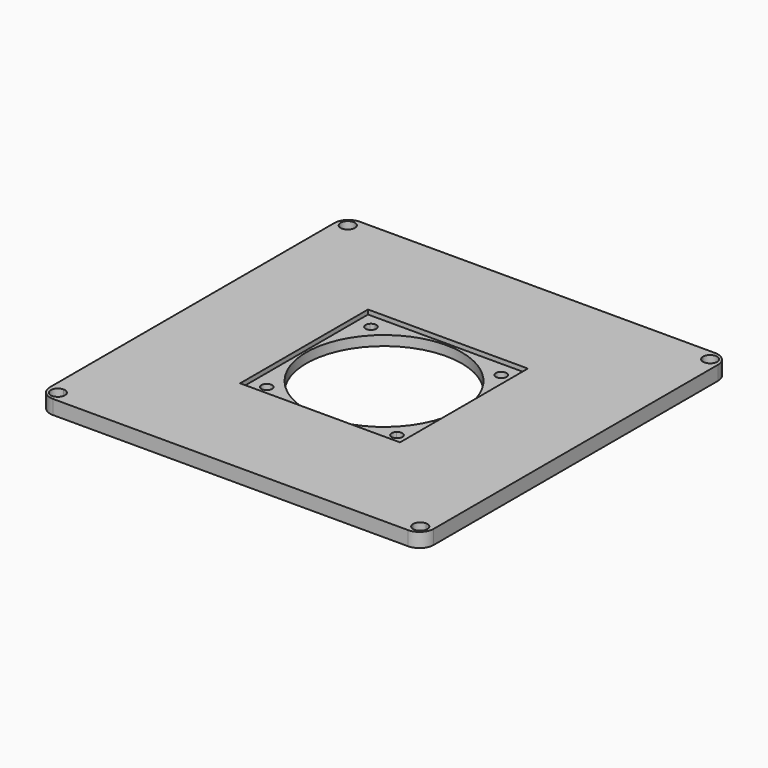
from build123d import *

# Parameters (mm, degrees)
F0_W             = 137.16
F0_H             = 137.16
F1_DEPTH         = 5.08
F2_R             = 5.08
F3_R             = 27.78125
F4_DEPTH         = 5.08
F5_W             = 57.15
F5_H             = 57.15
F6_DEPTH         = 1.5875
F8_DEPTH         = 3.4925
F8_COPIES_COUNT  = 4
F11_DEPTH        = 1.27
F11_COPIES_COUNT = 4
F13_DEPTH        = 5.08


# Not quite as in the source:
# - a pattern or mirror of a feature is missing from the dataset's text; its kind, count and spacing are read off the source's solid


with BuildPart() as f1:
    # F0 (on Top) → F1 (new body)
    with BuildSketch(Plane.XY):
        Rectangle(F0_W, F0_H)
    extrude(amount=F1_DEPTH)

    # F2
    f2_edges = [f1.edges().sort_by_distance(p)[0] for p in [
        (-68.58, -68.58, 2.54),
        (68.58, -68.58, 2.54),
        (68.58, 68.58, 2.54),
        (-68.58, 68.58, 2.54),
    ]]
    fillet(f2_edges, radius=F2_R)

    # F3 (on face) → F4 (cut, through all)
    with BuildSketch(Plane.XY.offset(5.08)):
        Circle(F3_R)
    extrude(amount=-F4_DEPTH, mode=Mode.SUBTRACT)

    # F5 (on face) → F6 (cut)
    with BuildSketch(Plane.XY.offset(5.08)):
        Rectangle(F5_W, F5_H)
    extrude(amount=-F6_DEPTH, mode=Mode.SUBTRACT)

    # F7 (on face) → F8 (cut, through all)
    with BuildSketch(Plane.XY.offset(3.4925)):
        with BuildLine():
            Line((21.9296104704, 21.9296104704), (24.6236873067, 24.6236873067))
            ThreePointArc((24.6236873067, 24.6236873067), (21.9296104704, 24.6236873067), (21.9296104704, 21.9296104704))
        make_face()
        with BuildLine():
            ThreePointArc((25.1816488886, 23.2766488886), (25.036639398, 24.0056608272), (24.6236873067, 24.6236873067))
            Line((24.6236873067, 24.6236873067), (21.9296104704, 21.9296104704))
            ThreePointArc((21.9296104704, 21.9296104704), (24.0056608272, 21.5166583791), (25.1816488886, 23.2766488886))
        make_face()
    f8 = extrude(amount=-F8_DEPTH, mode=Mode.SUBTRACT)

    # F8_copies: F8 ×4 about axis
    f8_copies_axis = Axis((0, 0, 0), (0, 0, 1))
    for i in range(1, F8_COPIES_COUNT):
        add(f8.rotate(f8_copies_axis, i * 360 / F8_COPIES_COUNT), mode=Mode.SUBTRACT)

    # F10 (on face) → F11 (cut)
    with BuildSketch(Plane(origin=(0, 0, 0), x_dir=(1, 0, 0), z_dir=(0, 0, -1))):
        Polygon((27.0866488886, 23.2766488886), (25.1816488886, 26.576205677), (21.3716488886, 26.576205677), (19.4666488886, 23.2766488886), (21.3716488886, 19.9770921002), (25.1816488886, 19.9770921002), align=None)
    f11 = extrude(amount=-F11_DEPTH, mode=Mode.SUBTRACT)

    # F11_copies: F11 ×4 about axis
    f11_copies_axis = Axis((0, 0, 0), (0, 0, 1))
    for i in range(1, F11_COPIES_COUNT):
        add(f11.rotate(f11_copies_axis, i * 360 / F11_COPIES_COUNT), mode=Mode.SUBTRACT)

    # F12 (on face) → F13 (cut, through all)
    with BuildSketch(Plane.XY.offset(5.08)):
        with BuildLine():
            Line((-64.77, 64.77), (-62.23, 64.77))
            ThreePointArc((-62.23, 64.77), (-66.5660512242, 66.5660512242), (-64.77, 62.23))
            Line((-64.77, 62.23), (-64.77, 64.77))
        make_face()
        with BuildLine():
            ThreePointArc((-64.77, 62.23), (-62.9739487758, 62.9739487758), (-62.23, 64.77))
            Line((-62.23, 64.77), (-64.77, 64.77))
            Line((-64.77, 64.77), (-64.77, 62.23))
        make_face()
        with BuildLine():
            Line((-64.77, -64.77), (-64.77, -62.23))
            ThreePointArc((-64.77, -62.23), (-66.5660512242, -66.5660512242), (-62.23, -64.77))
            Line((-62.23, -64.77), (-64.77, -64.77))
        make_face()
        with BuildLine():
            ThreePointArc((-62.23, -64.77), (-62.9739487758, -62.9739487758), (-64.77, -62.23))
            Line((-64.77, -62.23), (-64.77, -64.77))
            Line((-64.77, -64.77), (-62.23, -64.77))
        make_face()
        with BuildLine():
            ThreePointArc((67.31, -64.77), (66.5660512242, -62.9739487758), (64.77, -62.23))
            Line((64.77, -62.23), (64.77, -64.77))
            Line((64.77, -64.77), (62.23, -64.77))
            ThreePointArc((62.23, -64.77), (64.77, -67.31), (67.31, -64.77))
        make_face()
        with BuildLine():
            Line((64.77, -64.77), (64.77, -62.23))
            ThreePointArc((64.77, -62.23), (62.9739487758, -62.9739487758), (62.23, -64.77))
            Line((62.23, -64.77), (64.77, -64.77))
        make_face()
        with BuildLine():
            Line((64.77, 64.77), (62.23, 64.77))
            ThreePointArc((62.23, 64.77), (62.9739487758, 62.9739487758), (64.77, 62.23))
            Line((64.77, 62.23), (64.77, 64.77))
        make_face()
        with BuildLine():
            ThreePointArc((67.31, 64.77), (64.77, 67.31), (62.23, 64.77))
            Line((62.23, 64.77), (64.77, 64.77))
            Line((64.77, 64.77), (64.77, 62.23))
            ThreePointArc((64.77, 62.23), (66.5660512242, 62.9739487758), (67.31, 64.77))
        make_face()
    extrude(amount=-F13_DEPTH, mode=Mode.SUBTRACT)


solid = f1.part
